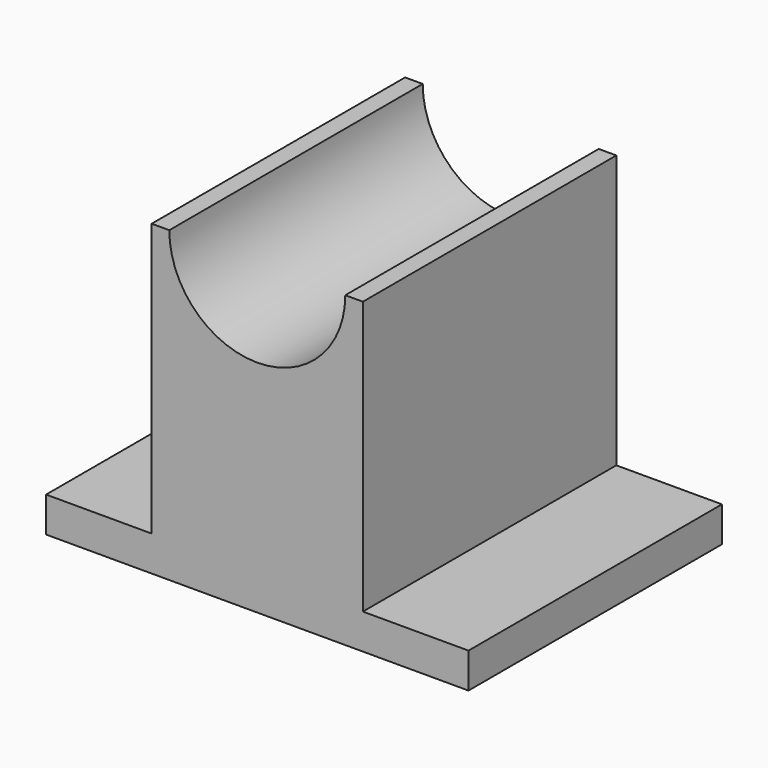
from build123d import *

# Parameters (mm, degrees)
F1_DEPTH = 114.3
F3_DEPTH = 114.301


# Not quite as in the source:
# - ends of sketch curves that miss each other by under 0.0002 mm in the source are joined


with BuildPart() as f1:
    # F0 (on Front) → F1 (new body)
    with BuildSketch(Plane.XZ):
        Polygon((-76.2, 0), (0, 0), (76.2, 0), (76.2, 12.7), (38.1, 12.7), (38.1, 111.125), (-38.1, 111.125), (-38.1, 12.7), (-76.2, 12.7), align=None)
    extrude(amount=F1_DEPTH)

    # F2 (on face) → F3 (cut, through all)
    with BuildSketch(Plane.XZ.offset(114.3)):
        with BuildLine():
            Line((0, 111.125), (-31.75, 111.125))
            ThreePointArc((-31.75, 111.125), (2.0181e-06, 79.3749959638), (31.75, 111.125))
            Line((31.75, 111.125), (0, 111.125))
        make_face()
    extrude(amount=-F3_DEPTH, mode=Mode.SUBTRACT)


solid = f1.part
